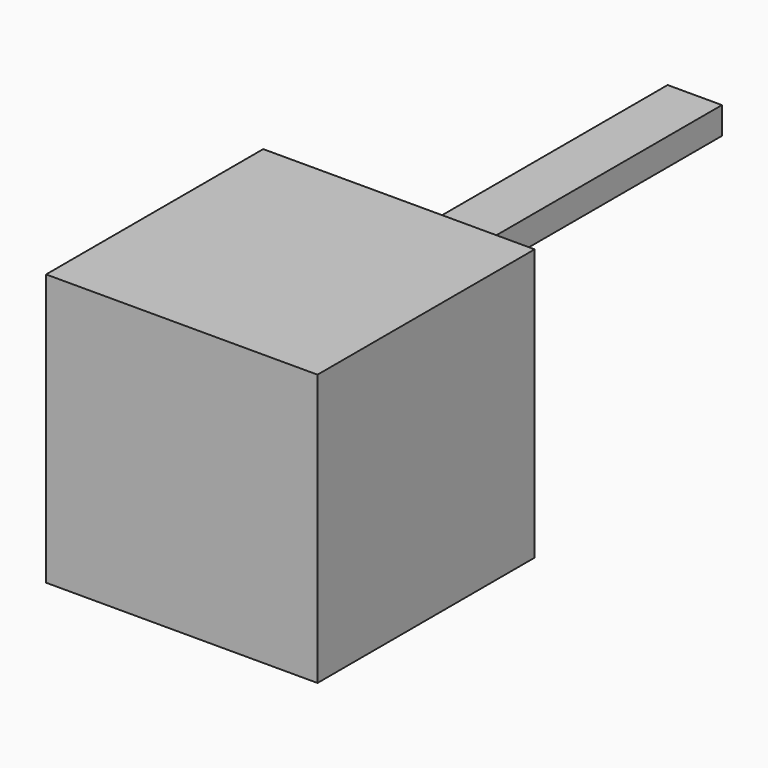
from build123d import *

# Parameters (mm, degrees)
F1_W     = 12.7
F1_H     = 12.7
F2_DEPTH = 6.35
F4_W     = 2.54
F4_H     = 1.27


# Not quite as in the source:
# - a variable given as a bare number and used for a length is read in inches; the dataset says mm whatever the document's units were


with BuildPart() as f2:
    # F1 (on Front) → F2 (new body, symmetric)
    with BuildSketch(Plane.XZ):
        Rectangle(F1_W, F1_H)
    extrude(amount=F2_DEPTH, both=True)


with BuildPart() as f5:
    # F5: sweep along a path in F3
    with BuildLine(Plane.YZ) as f5_path:
        Line((6.35, 2.9724712949), (23.6533820465, 2.9724712949))
    # F4 (on face) → F5 (sweep)
    with BuildSketch(Plane(origin=(0, 6.35, 0), x_dir=(-1, 0, 0), z_dir=(0, 1, 0))):
        with Locations((0, 2.9724712949)):
            Rectangle(F4_W, F4_H)
    sweep(path=f5_path.line)


solid = Compound([f2.part, f5.part])
